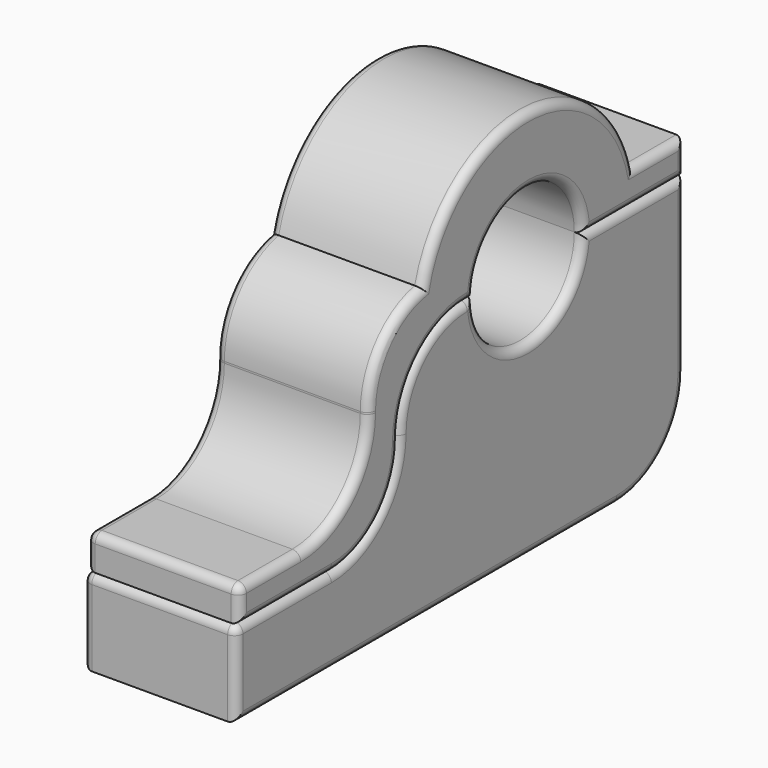
from build123d import *

# Parameters (mm, degrees)
F1_DEPTH    = 9
F2_R        = 5
F3_R        = 0.5
F4_DEPTH    = 9
F5_T1_DEPTH = 9
F5_T3_DEPTH = 9
F5_T5_DEPTH = 33.4948974279
F5_T7_DEPTH = 34
F6_T1_DEPTH = 9
F6_T4_ANGLE = 90
F6_T6_ANGLE = 90
F7_T1_DEPTH = 9
F7_T4_ANGLE = 90
F7_T6_ANGLE = 90
F8_R        = 0.5


# Not quite as in the source:
# - a fillet or chamfer that OpenCascade refuses, or shapes differently, is made with other operations: its cross-section is extruded or revolved along the edge and cut away or added


with BuildPart() as f1:
    # F0 (on Right) → F1 (new body)
    with BuildSketch(Plane.YZ):
        with BuildLine():
            Line((11.5, 12), (4, 12))
            ThreePointArc((4, 12), (0, 8), (-4, 12))
            Line((-4, 12), (-9.5, 12))
            Line((-9.5, 12), (-9.5, 2))
            Line((-9.5, 2), (-21.2459666924, 2))
            Line((-21.2459666924, 2), (-21.5, 2))
            Line((-21.5, 2), (-21.5, 0))
            Line((-21.5, 0), (-21.5, -3))
            Line((-21.5, -3), (11.5, -3))
            Line((11.5, -3), (11.5, 12))
        make_face()
    extrude(amount=F1_DEPTH)

    # F2
    f2_edges = [f1.edges().sort_by_distance(p)[0] for p in [
        (4.5, -9.5, 2),
    ]]
    fillet(f2_edges, radius=F2_R)

    # F3
    f3_edges = [f1.edges().sort_by_distance(p)[0] for p in [
        (0, -9.5, 9.5),
        (0, -10.964466, 3.464466),
        (0, -6.75, 12),
        (0, -18, 2),
        (0, 0, 8),
        (0, -21.5, -0.5),
        (0, 7.75, 12),
        (0, -5, -3),
        (0, 11.5, 4.5),
        (9, -9.5, 9.5),
        (9, -10.964466, 3.464466),
        (9, -6.75, 12),
        (9, -18, 2),
        (9, 0, 8),
        (9, -21.5, -0.5),
        (9, 7.75, 12),
        (9, -5, -3),
        (9, 11.5, 4.5),
        (4.5, -21.5, 2),
    ]]
    fillet(f3_edges, radius=F3_R)

    # F6: fillet of radius 5 on 1 edges, made by hand

    # F6_s2 → F6_t1 (cut)
    with BuildSketch(Plane.YZ):
        with BuildLine():
            ThreePointArc((-9.5, 7), (-8.0355339059, 10.5355339059), (-4.5, 12))
            Line((-4.5, 12), (-9.5, 12))
            Line((-9.5, 12), (-9.5, 7))
        make_face()
    extrude(amount=F6_T1_DEPTH, mode=Mode.SUBTRACT)

    # F6_s3 → F6_t4 (revolve, cut)
    with BuildSketch(Plane.XY.offset(7)):
        with BuildLine():
            ThreePointArc((0, -9), (0.1464466094, -9.3535533906), (0.5, -9.5))
            Line((0.5, -9.5), (0, -9.5))
            Line((0, -9.5), (0, -9))
        make_face()
    revolve(axis=Axis((0, -4.5, 7), (-1, 0, 0)), revolution_arc=F6_T4_ANGLE, mode=Mode.SUBTRACT)

    # F6_s5 → F6_t6 (revolve, cut)
    with BuildSketch(Plane.XZ.offset(4.5)):
        with BuildLine():
            ThreePointArc((9, 11.5), (8.8535533906, 11.8535533906), (8.5, 12))
            Line((8.5, 12), (9, 12))
            Line((9, 12), (9, 11.5))
        make_face()
    revolve(axis=Axis((9, -4.5, 7), (1, 0, 0)), revolution_arc=F6_T6_ANGLE, mode=Mode.SUBTRACT)

    # F7: fillet of radius 5 on 1 edges, made by hand

    # F7_s2 → F7_t1 (cut)
    with BuildSketch(Plane.YZ):
        with BuildLine():
            ThreePointArc((11.5, 2), (10.0355339059, -1.5355339059), (6.5, -3))
            Line((6.5, -3), (11.5, -3))
            Line((11.5, -3), (11.5, 2))
        make_face()
    extrude(amount=F7_T1_DEPTH, mode=Mode.SUBTRACT)

    # F7_s3 → F7_t4 (revolve, cut)
    with BuildSketch(Plane.XY.offset(2)):
        with BuildLine():
            ThreePointArc((0, 11), (0.1464466094, 11.3535533906), (0.5, 11.5))
            Line((0.5, 11.5), (0, 11.5))
            Line((0, 11.5), (0, 11))
        make_face()
    revolve(axis=Axis((0, 6.5, 2), (-1, 0, 0)), revolution_arc=F7_T4_ANGLE, mode=Mode.SUBTRACT)

    # F7_s5 → F7_t6 (revolve, cut)
    with BuildSketch(Plane.XZ.offset(-6.5)):
        with BuildLine():
            ThreePointArc((9, -2.5), (8.8535533906, -2.8535533906), (8.5, -3))
            Line((8.5, -3), (9, -3))
            Line((9, -3), (9, -2.5))
        make_face()
    revolve(axis=Axis((9, 6.5, 2), (1, 0, 0)), revolution_arc=F7_T6_ANGLE, mode=Mode.SUBTRACT)


with BuildPart() as f4:
    # F0 (on Right) → F4 (new body)
    with BuildSketch(Plane.YZ):
        with BuildLine():
            ThreePointArc((-4, 12), (0, 16), (4, 12))
            Line((4, 12), (11.5, 12))
            Line((11.5, 12), (11.5, 14))
            Line((11.5, 14), (7.7459666924, 14))
            ThreePointArc((7.7459666924, 14), (0, 20), (-7.7459666924, 14))
            Line((-7.7459666924, 14), (-11.7459666924, 14))
            Line((-11.7459666924, 14), (-11.7459666924, 4))
            Line((-11.7459666924, 4), (-21.2459666924, 4))
            Line((-21.2459666924, 4), (-21.2459666924, 2))
            Line((-21.2459666924, 2), (-9.5, 2))
            Line((-9.5, 2), (-9.5, 12))
            Line((-9.5, 12), (-4, 12))
        make_face()
    extrude(amount=F4_DEPTH)

    # F5: fillet of radius 5 on 4 edges, made by hand

    # F5_s2 → F5_t1 (join)
    with BuildSketch(Plane.YZ):
        with BuildLine():
            ThreePointArc((-11.7459666924, 9), (-13.2104327865, 5.4644660941), (-16.7459666924, 4))
            Line((-16.7459666924, 4), (-11.7459666924, 4))
            Line((-11.7459666924, 4), (-11.7459666924, 9))
        make_face()
    extrude(amount=F5_T1_DEPTH)

    # F5_s4 → F5_t3 (join)
    with BuildSketch(Plane.YZ):
        with BuildLine():
            ThreePointArc((-4.5, 12), (-8.0355339059, 10.5355339059), (-9.5, 7))
            Line((-9.5, 7), (-9.5, 12))
            Line((-9.5, 12), (-4.5, 12))
        make_face()
    extrude(amount=F5_T3_DEPTH)

    # F5_s6 → F5_t5 (cut)
    with BuildSketch(Plane.YZ.offset(-12.2474487139)):
        with BuildLine():
            ThreePointArc((-7.7459666924, 14), (-10.6189500386, 12.2632981746), (-11.7459666924, 9.1010205144))
            Line((-11.7459666924, 9.1010205144), (-11.7459666924, 14))
            Line((-11.7459666924, 14), (-7.7459666924, 14))
        make_face()
    extrude(amount=F5_T5_DEPTH, mode=Mode.SUBTRACT)

    # F5_s8 → F5_t7 (cut)
    with BuildSketch(Plane.YZ.offset(-12.5)):
        with BuildLine():
            ThreePointArc((-9.5, 7), (-10.9644660941, 3.4644660941), (-14.5, 2))
            Line((-14.5, 2), (-9.5, 2))
            Line((-9.5, 2), (-9.5, 7))
        make_face()
    extrude(amount=F5_T7_DEPTH, mode=Mode.SUBTRACT)

    # F8
    f8_edges = [f4.edges().sort_by_distance(p)[0] for p in [
        (9, -8.035534, 10.535534),
        (9, -10.964466, 3.464466),
        (9, -17.872983, 2),
        (9, -21.245967, 3),
        (9, -18.995967, 4),
        (9, -13.210433, 5.464466),
        (9, -11.745967, 9.05051),
        (9, -10.61895, 12.263298),
        (9, 0, 20),
        (9, 9.622983, 14),
        (9, 11.5, 13),
        (9, 7.75, 12),
        (9, 0, 16),
        (9, -4.25, 12),
        (0, -8.035534, 10.535534),
        (0, -10.964466, 3.464466),
        (0, -17.872983, 2),
        (0, -21.245967, 3),
        (0, -18.995967, 4),
        (0, -13.210433, 5.464466),
        (0, -11.745967, 9.05051),
        (0, -10.61895, 12.263298),
        (0, 0, 20),
        (0, 9.622983, 14),
        (0, 11.5, 13),
        (0, 7.75, 12),
        (0, 0, 16),
        (0, -4.25, 12),
        (4.5, -21.245967, 4),
        (4.5, -16.745967, 4),
    ]]
    fillet(f8_edges, radius=F8_R)


solid = Compound([f1.part, f4.part])
